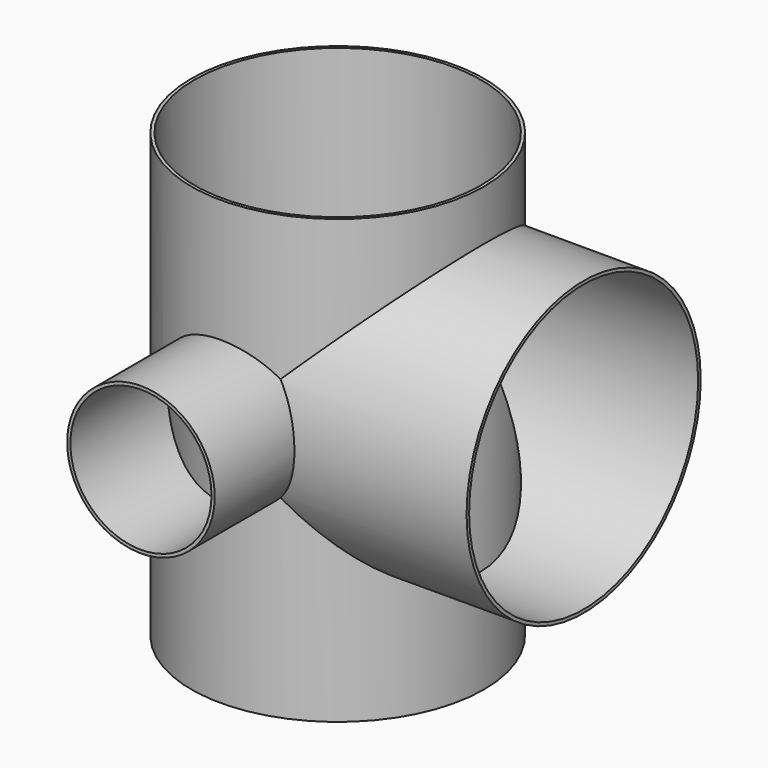
from build123d import *

# Parameters (mm, degrees)
F0_R      = 75.565
F1_DEPTH  = 101.6
F2_DEPTH  = 127
F3_R      = 38.1
F4_DEPTH  = 127
F5_R      = 75.565
F6_DEPTH  = 127
F7_R      = 73.914
F8_DEPTH  = 228.6010001
F9_R      = 73.914
F10_DEPTH = 127.001
F11_R     = 36.449
F12_DEPTH = 62.6989799529


with BuildPart() as f1:
    # F0 (on Top) → F1 (new body)
    with BuildSketch(Plane.XY):
        Circle(F0_R)
    extrude(amount=F1_DEPTH)

    # F0 (on Top) → F2 (join)
    with BuildSketch(Plane.XY):
        Circle(F0_R)
    extrude(amount=-F2_DEPTH)

    # F3 (on Front) → F4 (join)
    with BuildSketch(Plane.XZ):
        Circle(F3_R)
    extrude(amount=F4_DEPTH)

    # F5 (on Right) → F6 (join)
    with BuildSketch(Plane.YZ):
        Circle(F5_R)
    extrude(amount=F6_DEPTH)

    # F7 (on face) → F8 (cut, through all)
    with BuildSketch(Plane.XY.offset(101.6)):
        Circle(F7_R)
    extrude(amount=-F8_DEPTH, mode=Mode.SUBTRACT)

    # F9 (on face) → F10 (cut, through all)
    with BuildSketch(Plane.YZ.offset(127)):
        Circle(F9_R)
    extrude(amount=-F10_DEPTH, mode=Mode.SUBTRACT)

    # F11 (on face) → F12 (cut, through all)
    with BuildSketch(Plane.XZ.offset(127)):
        Circle(F11_R)
    extrude(amount=-F12_DEPTH, mode=Mode.SUBTRACT)


solid = f1.part
